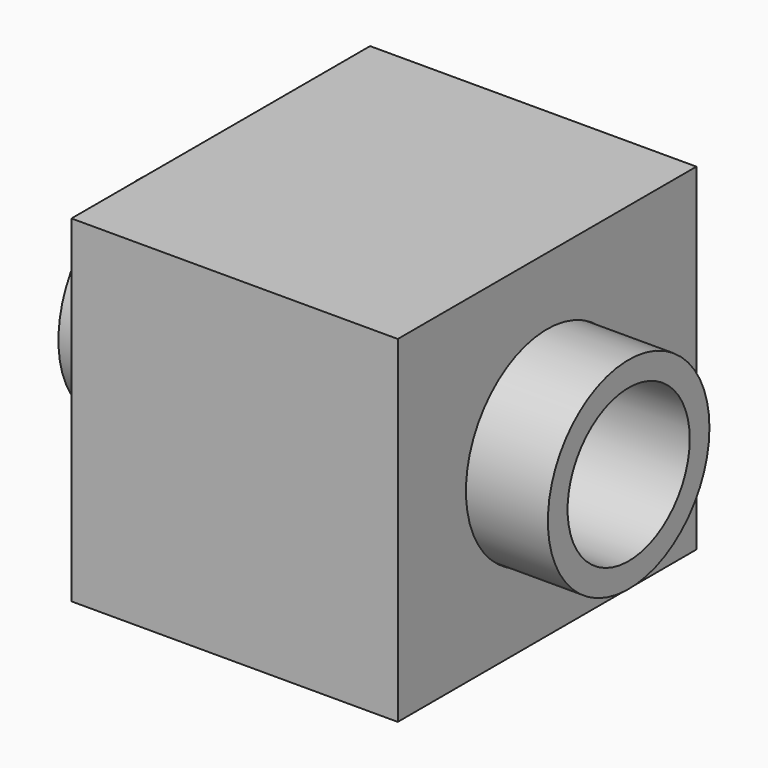
from build123d import *

# Parameters (mm, degrees)
F0_W     = 116.2151992321
F0_H     = 104.9675941467
F0_R     = 31.5798235418
F1_DEPTH = 50.8
F2_R     = 31.4378135925
F2_R_2   = 23.771453385
F3_DEPTH = 76.2


# Not quite as in the source:
# - a feature of the source that left no trace in its solid (it failed there, or was rolled back) is left out


with BuildPart() as f1:
    # F0 (on Right) → F1 (new body, symmetric)
    with BuildSketch(Plane.YZ):
        Rectangle(F0_W, F0_H)
        Circle(F0_R, mode=Mode.SUBTRACT)
    extrude(amount=F1_DEPTH, both=True)


with BuildPart() as f3:
    # F2 (on Right) → F3 (new body, symmetric)
    with BuildSketch(Plane.YZ):
        Circle(F2_R)
        Circle(F2_R_2, mode=Mode.SUBTRACT)
    extrude(amount=F3_DEPTH, both=True)


solid = Compound([f1.part, f3.part])
